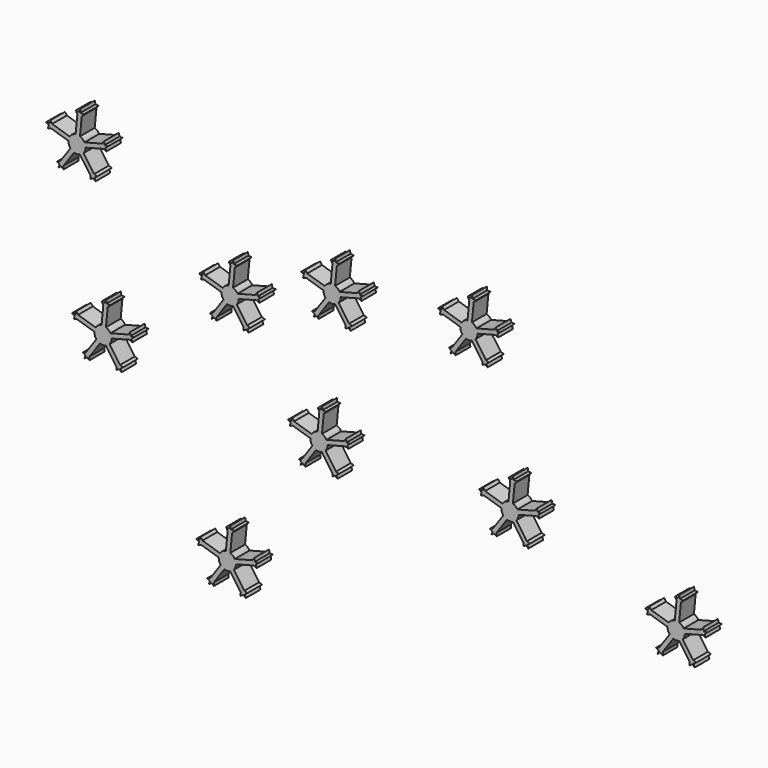
from build123d import *

# Parameters (mm, degrees)
F1_DEPTH = 6.35


# Not quite as in the source:
# - a length typed as a fraction of an inch, garbled in the dataset ("3 / 203.2 mm" for 3/8 in), is restored
# - a feature names something its author has since deleted; it is built from what else it names


with BuildPart() as f1:
    # F0 (on Front) → F1 (new body)
    with BuildSketch(Plane.XZ):
        with BuildLine():
            Line((21.2604275488, -3.1095474934), (20.6556292887, -9.4079404551))
            ThreePointArc((20.6556292887, -9.4079404551), (19.4937557739, -9.8666915905), (18.6236292887, -10.7629519146))
            Line((18.6236292887, -10.7629519146), (12.576675601, -8.900188931))
            Line((12.576675601, -8.900188931), (12.1280131248, -10.3566497037))
            Line((12.1280131248, -10.3566497037), (18.1749668126, -12.2194126873))
            ThreePointArc((18.1749668126, -12.2194126873), (18.3341547138, -13.3009294793), (18.8741556679, -14.2514126873))
            Line((18.8741556679, -14.2514126873), (15.2537081429, -19.4406221217))
            Line((15.2537081429, -19.4406221217), (16.5035738394, -20.3126380279))
            Line((16.5035738394, -20.3126380279), (20.1240213644, -15.1234285936))
            ThreePointArc((20.1240213644, -15.1234285936), (21.1400213644, -15.302786315), (22.1560213644, -15.1234285936))
            Line((22.1560213644, -15.1234285936), (25.7764688895, -20.3126380279))
            Line((25.7764688895, -20.3126380279), (27.026334586, -19.4406221217))
            Line((27.026334586, -19.4406221217), (23.4058870609, -14.2514126873))
            ThreePointArc((23.4058870609, -14.2514126873), (23.9249424171, -13.3597811887), (24.107332834, -12.3443212298))
            Line((24.107332834, -12.3443212298), (30.2273350961, -10.7377387866))
            Line((30.2273350961, -10.7377387866), (29.8403759052, -9.2636836369))
            Line((29.8403759052, -9.2636836369), (23.720373643, -10.87026608))
            ThreePointArc((23.720373643, -10.87026608), (23.0627291406, -10.0753265221), (22.1726513719, -9.5536113146))
            Line((22.1726513719, -9.5536113146), (22.7774496319, -3.2552183529))
            Line((22.7774496319, -3.2552183529), (21.2604275488, -3.1095474934))
        make_face()
        Polygon((12.1280131248, -10.3566497037), (12.576675601, -8.900188931), (11.9083695148, -8.0093797881), (11.5805188378, -9.0736578943), (10.4671907922, -9.0476845099), (11.4021389343, -9.6527018033), (11.0742882573, -10.7169799096), align=None)
        Polygon((20.6949701578, -2.1501670916), (21.2604275488, -3.1095474934), (22.7774496319, -3.2552183529), (23.5151386713, -2.4209715683), (22.4066161069, -2.3145265557), (22.2074849753, -1.2188534252), (21.8034927222, -2.2566121042), align=None)
        Polygon((30.4565886994, -8.3360874916), (29.8403759052, -9.2636836369), (30.2273350961, -10.7377387866), (31.232289885, -11.2175498836), (30.9624783419, -10.1371080538), (31.8394937863, -9.4508160411), (30.7264002425, -9.4165293214), align=None)
        Polygon((28.0786650957, -19.8049719039), (27.026334586, -19.4406221217), (25.7764688895, -20.3126380279), (25.75514866, -21.4260542633), (26.6684530327, -20.7888530485), (27.5300695705, -21.4943792401), (27.165360723, -20.4421731187), align=None)
        Polygon((16.5035738394, -20.3126380279), (15.2537081429, -19.4406221217), (14.2013746901, -19.8049634034), (15.1146790628, -20.4421646183), (14.7499518509, -21.4943643741), (15.6115807023, -20.7888532206), (16.524885075, -21.4260544355), align=None)
    extrude(amount=F1_DEPTH)


with BuildPart() as f1b:
    # F0 (on Front) → F1, piece 2 (new body)
    with BuildSketch(Plane.XZ):
        with BuildLine():
            Line((-25.9454713619, -7.3767473896), (-26.550269622, -13.6751403513))
            ThreePointArc((-26.550269622, -13.6751403513), (-27.7121431369, -14.1338914867), (-28.582269622, -15.0301518109))
            Line((-28.582269622, -15.0301518109), (-34.6292233098, -13.1673888273))
            Line((-34.6292233098, -13.1673888273), (-35.0778857859, -14.6238496))
            Line((-35.0778857859, -14.6238496), (-29.0309320981, -16.4866125836))
            ThreePointArc((-29.0309320981, -16.4866125836), (-28.8717441969, -17.5681293756), (-28.3317432428, -18.5186125836))
            Line((-28.3317432428, -18.5186125836), (-31.9521907679, -23.707822018))
            Line((-31.9521907679, -23.707822018), (-30.7023250714, -24.5798379242))
            Line((-30.7023250714, -24.5798379242), (-27.0818775463, -19.3906284899))
            ThreePointArc((-27.0818775463, -19.3906284899), (-26.0658775463, -19.5699862113), (-25.0498775463, -19.3906284899))
            Line((-25.0498775463, -19.3906284899), (-21.4294300213, -24.5798379242))
            Line((-21.4294300213, -24.5798379242), (-20.1795643248, -23.707822018))
            Line((-20.1795643248, -23.707822018), (-23.8000118498, -18.5186125836))
            ThreePointArc((-23.8000118498, -18.5186125836), (-23.2809564936, -17.6269810849), (-23.0985660768, -16.6115211261))
            Line((-23.0985660768, -16.6115211261), (-16.9785638147, -15.0049386829))
            Line((-16.9785638147, -15.0049386829), (-17.3655230056, -13.5308835331))
            Line((-17.3655230056, -13.5308835331), (-23.4855252677, -15.1374659763))
            ThreePointArc((-23.4855252677, -15.1374659763), (-24.1431697701, -14.3425264184), (-25.0332475389, -13.8208112109))
            Line((-25.0332475389, -13.8208112109), (-24.4284492788, -7.5224182492))
            Line((-24.4284492788, -7.5224182492), (-25.9454713619, -7.3767473896))
        make_face()
        Polygon((-19.1272338151, -24.0721718001), (-20.1795643248, -23.707822018), (-21.4294300213, -24.5798379242), (-21.4507502507, -25.6932541596), (-20.5374458781, -25.0560529447), (-19.6758293402, -25.7615791364), (-20.0405381878, -24.709373015), align=None)
        Polygon((-30.7023250714, -24.5798379242), (-31.9521907679, -23.707822018), (-33.0045242206, -24.0721632997), (-32.0912198479, -24.7093645145), (-32.4559470599, -25.7615642704), (-31.5943182084, -25.0560531169), (-30.6810138358, -25.6932543318), align=None)
        Polygon((-35.0778857859, -14.6238496), (-34.6292233098, -13.1673888273), (-35.2975293959, -12.2765796844), (-35.625380073, -13.3408577906), (-36.7387081186, -13.3148844062), (-35.8037599765, -13.9199016996), (-36.1316106535, -14.9841798058), align=None)
        Polygon((-26.5109287529, -6.4173669878), (-25.9454713619, -7.3767473896), (-24.4284492788, -7.5224182492), (-23.6907602395, -6.6881714645), (-24.7992828039, -6.5817264519), (-24.9984139354, -5.4860533215), (-25.4024061886, -6.5238120004), align=None)
        Polygon((-16.7493102114, -12.6032873879), (-17.3655230056, -13.5308835331), (-16.9785638147, -15.0049386829), (-15.9736090258, -15.4847497799), (-16.2434205689, -14.4043079501), (-15.3664051245, -13.7180159374), (-16.4794986683, -13.6837292177), align=None)
    extrude(amount=F1_DEPTH)


with BuildPart() as f1c:
    # F0 (on Front) → F1, piece 3 (new body)
    with BuildSketch(Plane.XZ):
        with BuildLine():
            Line((-61.1498726017, -19.3782487859), (-61.7546708618, -25.6766417476))
            ThreePointArc((-61.7546708618, -25.6766417476), (-62.9165443766, -26.135392883), (-63.7866708618, -27.0316532072))
            Line((-63.7866708618, -27.0316532072), (-69.8336245495, -25.1688902236))
            Line((-69.8336245495, -25.1688902236), (-70.2822870257, -26.6253509963))
            Line((-70.2822870257, -26.6253509963), (-64.2353333379, -28.4881139799))
            ThreePointArc((-64.2353333379, -28.4881139799), (-64.0761454367, -29.5696307719), (-63.5361444826, -30.5201139799))
            Line((-63.5361444826, -30.5201139799), (-67.1565920076, -35.7093234143))
            Line((-67.1565920076, -35.7093234143), (-65.9067263111, -36.5813393205))
            Line((-65.9067263111, -36.5813393205), (-62.2862787861, -31.3921298862))
            ThreePointArc((-62.2862787861, -31.3921298862), (-61.2702787861, -31.5714876076), (-60.2542787861, -31.3921298862))
            Line((-60.2542787861, -31.3921298862), (-56.633831261, -36.5813393205))
            Line((-56.633831261, -36.5813393205), (-55.3839655645, -35.7093234143))
            Line((-55.3839655645, -35.7093234143), (-59.0044130896, -30.5201139799))
            ThreePointArc((-59.0044130896, -30.5201139799), (-58.4853577334, -29.6284824812), (-58.3029673166, -28.6130225224))
            Line((-58.3029673166, -28.6130225224), (-52.1829650544, -27.0064400792))
            Line((-52.1829650544, -27.0064400792), (-52.5699242453, -25.5323849294))
            Line((-52.5699242453, -25.5323849294), (-58.6899265075, -27.1389673726))
            ThreePointArc((-58.6899265075, -27.1389673726), (-59.3475710099, -26.3440278147), (-60.2376487786, -25.8223126072))
            Line((-60.2376487786, -25.8223126072), (-59.6328505186, -19.5239196455))
            Line((-59.6328505186, -19.5239196455), (-61.1498726017, -19.3782487859))
        make_face()
        Polygon((-51.9537114511, -24.6047887842), (-52.5699242453, -25.5323849294), (-52.1829650544, -27.0064400792), (-51.1780102656, -27.4862511762), (-51.4478218086, -26.4058093464), (-50.5708063642, -25.7195173337), (-51.683899908, -25.685230614), align=None)
        Polygon((-61.7153299927, -18.4188683841), (-61.1498726017, -19.3782487859), (-59.6328505186, -19.5239196455), (-58.8951614792, -18.6896728608), (-60.0036840436, -18.5832278482), (-60.2028151752, -17.4875547178), (-60.6068074283, -18.5253133967), align=None)
        Polygon((-70.2822870257, -26.6253509963), (-69.8336245495, -25.1688902236), (-70.5019306357, -24.2780810807), (-70.8297813127, -25.3423591869), (-71.9431093583, -25.3163858025), (-71.0081612162, -25.9214030959), (-71.3360118933, -26.9856812021), align=None)
        Polygon((-54.3316350549, -36.0736731964), (-55.3839655645, -35.7093234143), (-56.633831261, -36.5813393205), (-56.6551514905, -37.6947555559), (-55.7418471178, -37.057554341), (-54.88023058, -37.7630805327), (-55.2449394275, -36.7108744113), align=None)
        Polygon((-65.9067263111, -36.5813393205), (-67.1565920076, -35.7093234143), (-68.2089254604, -36.073664696), (-67.2956210877, -36.7108659108), (-67.6603482997, -37.7630656667), (-66.7987194482, -37.0575545132), (-65.8854150755, -37.6947557281), align=None)
    extrude(amount=F1_DEPTH)


with BuildPart() as f1d:
    # F0 (on Front) → F1, piece 4 (new body)
    with BuildSketch(Plane.XZ):
        with BuildLine():
            Line((-113.95647353, 9.4253530751), (-114.5612717901, 3.1269601134))
            ThreePointArc((-114.5612717901, 3.1269601134), (-115.723145305, 2.668208978), (-116.5932717901, 1.7719486538))
            Line((-116.5932717901, 1.7719486538), (-122.6402254779, 3.6347116374))
            Line((-122.6402254779, 3.6347116374), (-123.088887954, 2.1782508647))
            Line((-123.088887954, 2.1782508647), (-117.0419342662, 0.3154878811))
            ThreePointArc((-117.0419342662, 0.3154878811), (-116.882746365, -0.7660289109), (-116.3427454109, -1.7165121189))
            Line((-116.3427454109, -1.7165121189), (-119.9631929359, -6.9057215533))
            Line((-119.9631929359, -6.9057215533), (-118.7133272394, -7.7777374595))
            Line((-118.7133272394, -7.7777374595), (-115.0928797144, -2.5885280252))
            ThreePointArc((-115.0928797144, -2.5885280252), (-114.0768797144, -2.7678857466), (-113.0608797144, -2.5885280252))
            Line((-113.0608797144, -2.5885280252), (-109.4404321893, -7.7777374595))
            Line((-109.4404321893, -7.7777374595), (-108.1905664928, -6.9057215533))
            Line((-108.1905664928, -6.9057215533), (-111.8110140179, -1.7165121189))
            ThreePointArc((-111.8110140179, -1.7165121189), (-111.2919586617, -0.8248806202), (-111.1095682449, 0.1905793386))
            Line((-111.1095682449, 0.1905793386), (-104.9895659827, 1.7971617818))
            Line((-104.9895659827, 1.7971617818), (-105.3765251736, 3.2712169316))
            Line((-105.3765251736, 3.2712169316), (-111.4965274358, 1.6646344884))
            ThreePointArc((-111.4965274358, 1.6646344884), (-112.1541719382, 2.4595740463), (-113.044249707, 2.9812892538))
            Line((-113.044249707, 2.9812892538), (-112.4394514469, 9.2796822155))
            Line((-112.4394514469, 9.2796822155), (-113.95647353, 9.4253530751))
        make_face()
        Polygon((-114.521930921, 10.3847334769), (-113.95647353, 9.4253530751), (-112.4394514469, 9.2796822155), (-111.7017624075, 10.1139290002), (-112.8102849719, 10.2203740128), (-113.0094161035, 11.3160471432), (-113.4134083566, 10.2782884643), align=None)
        Polygon((-104.7603123795, 4.1988130768), (-105.3765251736, 3.2712169316), (-104.9895659827, 1.7971617818), (-103.9846111939, 1.3173506848), (-104.254422737, 2.3977925146), (-103.3774072925, 3.0840845273), (-104.4905008364, 3.118371247), align=None)
        Polygon((-123.088887954, 2.1782508647), (-122.6402254779, 3.6347116374), (-123.308531564, 4.5255207803), (-123.636382241, 3.4612426741), (-124.7497102866, 3.4872160585), (-123.8147621445, 2.8821987651), (-124.1426128216, 1.8179206589), align=None)
        Polygon((-118.7133272394, -7.7777374595), (-119.9631929359, -6.9057215533), (-121.0155263887, -7.270062835), (-120.102222016, -7.9072640498), (-120.466949228, -8.9594638057), (-119.6053203765, -8.2539526522), (-118.6920160038, -8.8911538671), align=None)
        Polygon((-107.1382359832, -7.2700713354), (-108.1905664928, -6.9057215533), (-109.4404321893, -7.7777374595), (-109.4617524188, -8.8911536949), (-108.5484480461, -8.25395248), (-107.6868315083, -8.9594786717), (-108.0515403558, -7.9072725503), align=None)
    extrude(amount=F1_DEPTH)


with BuildPart() as f1e:
    # F0 (on Front) → F1, piece 5 (new body)
    with BuildSketch(Plane.XZ):
        with BuildLine():
            Line((-105.0079462535, -45.6497373035), (-105.6127445136, -51.9481302652))
            ThreePointArc((-105.6127445136, -51.9481302652), (-106.7746180284, -52.4068814005), (-107.6447445136, -53.3031417247))
            Line((-107.6447445136, -53.3031417247), (-113.6916982013, -51.4403787411))
            Line((-113.6916982013, -51.4403787411), (-114.1403606775, -52.8968395138))
            Line((-114.1403606775, -52.8968395138), (-108.0934069897, -54.7596024974))
            ThreePointArc((-108.0934069897, -54.7596024974), (-107.9342190885, -55.8411192894), (-107.3942181344, -56.7916024974))
            Line((-107.3942181344, -56.7916024974), (-111.0146656594, -61.9808119318))
            Line((-111.0146656594, -61.9808119318), (-109.7647999629, -62.852827838))
            Line((-109.7647999629, -62.852827838), (-106.1443524379, -57.6636184037))
            ThreePointArc((-106.1443524379, -57.6636184037), (-105.1283524379, -57.8429761251), (-104.1123524379, -57.6636184037))
            Line((-104.1123524379, -57.6636184037), (-100.4919049128, -62.852827838))
            Line((-100.4919049128, -62.852827838), (-99.2420392163, -61.9808119318))
            Line((-99.2420392163, -61.9808119318), (-102.8624867414, -56.7916024974))
            ThreePointArc((-102.8624867414, -56.7916024974), (-102.3434313852, -55.8999709988), (-102.1610409683, -54.8845110399))
            Line((-102.1610409683, -54.8845110399), (-96.0410387062, -53.2779285967))
            Line((-96.0410387062, -53.2779285967), (-96.4279978971, -51.803873447))
            Line((-96.4279978971, -51.803873447), (-102.5480001593, -53.4104558901))
            ThreePointArc((-102.5480001593, -53.4104558901), (-103.2056446617, -52.6155163322), (-104.0957224304, -52.0938011247))
            Line((-104.0957224304, -52.0938011247), (-103.4909241704, -45.795408163))
            Line((-103.4909241704, -45.795408163), (-105.0079462535, -45.6497373035))
        make_face()
        Polygon((-105.5734036445, -44.6903569017), (-105.0079462535, -45.6497373035), (-103.4909241704, -45.795408163), (-102.753235131, -44.9611613784), (-103.8617576954, -44.8547163658), (-104.060888827, -43.7590432353), (-104.4648810801, -44.7968019143), align=None)
        Polygon((-114.1403606775, -52.8968395138), (-113.6916982013, -51.4403787411), (-114.3600042875, -50.5495695982), (-114.6878549645, -51.6138477044), (-115.8011830101, -51.58787432), (-114.866234868, -52.1928916134), (-115.194085545, -53.2571697197), align=None)
        Polygon((-95.8117851029, -50.8762773017), (-96.4279978971, -51.803873447), (-96.0410387062, -53.2779285967), (-95.0360839173, -53.7577396937), (-95.3058954604, -52.6772978639), (-94.428880016, -51.9910058512), (-95.5419735598, -51.9567191315), align=None)
        Polygon((-98.1897087066, -62.345161714), (-99.2420392163, -61.9808119318), (-100.4919049128, -62.852827838), (-100.5132251423, -63.9662440734), (-99.5999207696, -63.3290428586), (-98.7383042318, -64.0345690502), (-99.1030130793, -62.9823629288), align=None)
        Polygon((-109.7647999629, -62.852827838), (-111.0146656594, -61.9808119318), (-112.0669991122, -62.3451532135), (-111.1536947395, -62.9823544284), (-111.5184219514, -64.0345541842), (-110.6567931, -63.3290430307), (-109.7434887273, -63.9662442456), align=None)
    extrude(amount=F1_DEPTH)


with BuildPart() as f1f:
    # F0 (on Front) → F1, piece 6 (new body)
    with BuildSketch(Plane.XZ):
        Polygon((-62.6628538548, -99.3037869547), (-62.0973964638, -100.2631673565), (-60.5803743807, -100.408838216), (-59.8426853414, -99.5745914314), (-60.9512079057, -99.4681464188), (-61.1503390373, -98.3724732883), (-61.5543312905, -99.4102319673), align=None)
        Polygon((-52.9012353133, -105.4897073547), (-53.5174481075, -106.4173035), (-53.1304889165, -107.8913586497), (-52.1255341277, -108.3711697467), (-52.3953456708, -107.2907279169), (-51.5183302264, -106.6044359042), (-52.6314237702, -106.5701491845), align=None)
        Polygon((-55.279158917, -116.9585917669), (-56.3314894267, -116.5942419848), (-57.5813551232, -117.466257891), (-57.6026753526, -118.5796741264), (-56.6893709799, -117.9424729116), (-55.8277544421, -118.6479991032), (-56.1924632897, -117.5957929818), align=None)
        Polygon((-66.8542501732, -117.466257891), (-68.1041158697, -116.5942419848), (-69.1564493225, -116.9585832665), (-68.2431449498, -117.5957844814), (-68.6078721618, -118.6479842372), (-67.7462433103, -117.9424730837), (-66.8329389376, -118.5796742986), align=None)
        with BuildLine():
            Line((-62.0973964638, -100.2631673565), (-62.7021947239, -106.5615603182))
            ThreePointArc((-62.7021947239, -106.5615603182), (-63.8640682388, -107.0203114535), (-64.7341947239, -107.9165717777))
            Line((-64.7341947239, -107.9165717777), (-70.7811484117, -106.0538087941))
            Line((-70.7811484117, -106.0538087941), (-71.2298108878, -107.5102695668))
            Line((-71.2298108878, -107.5102695668), (-65.1828572, -109.3730325504))
            ThreePointArc((-65.1828572, -109.3730325504), (-65.0236692988, -110.4545493424), (-64.4836683447, -111.4050325504))
            Line((-64.4836683447, -111.4050325504), (-68.1041158697, -116.5942419848))
            Line((-68.1041158697, -116.5942419848), (-66.8542501732, -117.466257891))
            Line((-66.8542501732, -117.466257891), (-63.2338026482, -112.2770484567))
            ThreePointArc((-63.2338026482, -112.2770484567), (-62.2178026482, -112.4564061781), (-61.2018026482, -112.2770484567))
            Line((-61.2018026482, -112.2770484567), (-57.5813551232, -117.466257891))
            Line((-57.5813551232, -117.466257891), (-56.3314894267, -116.5942419848))
            Line((-56.3314894267, -116.5942419848), (-59.9519369517, -111.4050325504))
            ThreePointArc((-59.9519369517, -111.4050325504), (-59.4328815955, -110.5134010518), (-59.2504911787, -109.4979410929))
            Line((-59.2504911787, -109.4979410929), (-53.1304889165, -107.8913586497))
            Line((-53.1304889165, -107.8913586497), (-53.5174481075, -106.4173035))
            Line((-53.5174481075, -106.4173035), (-59.6374503696, -108.0238859431))
            ThreePointArc((-59.6374503696, -108.0238859431), (-60.295094872, -107.2289463852), (-61.1851726408, -106.7072311777))
            Line((-61.1851726408, -106.7072311777), (-60.5803743807, -100.408838216))
            Line((-60.5803743807, -100.408838216), (-62.0973964638, -100.2631673565))
        make_face()
        Polygon((-71.2298108878, -107.5102695668), (-70.7811484117, -106.0538087941), (-71.4494544978, -105.1629996512), (-71.7773051749, -106.2272777574), (-72.8906332204, -106.201304373), (-71.9556850783, -106.8063216664), (-72.2835357554, -107.8705997727), align=None)
    extrude(amount=F1_DEPTH)


with BuildPart() as f1g:
    # F0 (on Front) → F1, piece 7 (new body)
    with BuildSketch(Plane.XZ):
        Polygon((-31.0448287009, -52.8231685374), (-30.4793713099, -53.7825489392), (-28.9623492268, -53.9282197987), (-28.2246601875, -53.0939730141), (-29.3331827519, -52.9875280015), (-29.5323138834, -51.891854871), (-29.9363061366, -52.92961355), align=None)
        with BuildLine():
            Line((-30.4793713099, -53.7825489392), (-31.08416957, -60.0809419009))
            ThreePointArc((-31.08416957, -60.0809419009), (-32.2460430849, -60.5396930363), (-33.11616957, -61.4359533604))
            Line((-33.11616957, -61.4359533604), (-39.1631232578, -59.5731903768))
            Line((-39.1631232578, -59.5731903768), (-39.6117857339, -61.0296511496))
            Line((-39.6117857339, -61.0296511496), (-33.5648320461, -62.8924141332))
            ThreePointArc((-33.5648320461, -62.8924141332), (-33.4056441449, -63.9739309251), (-32.8656431908, -64.9244141332))
            Line((-32.8656431908, -64.9244141332), (-36.4860907159, -70.1136235675))
            Line((-36.4860907159, -70.1136235675), (-35.2362250194, -70.9856394738))
            Line((-35.2362250194, -70.9856394738), (-31.6157774943, -65.7964300394))
            ThreePointArc((-31.6157774943, -65.7964300394), (-30.5997774943, -65.9757877608), (-29.5837774943, -65.7964300394))
            Line((-29.5837774943, -65.7964300394), (-25.9633299693, -70.9856394738))
            Line((-25.9633299693, -70.9856394738), (-24.7134642728, -70.1136235675))
            Line((-24.7134642728, -70.1136235675), (-28.3339117978, -64.9244141332))
            ThreePointArc((-28.3339117978, -64.9244141332), (-27.8148564416, -64.0327826345), (-27.6324660248, -63.0173226756))
            Line((-27.6324660248, -63.0173226756), (-21.5124637627, -61.4107402325))
            Line((-21.5124637627, -61.4107402325), (-21.8994229536, -59.9366850827))
            Line((-21.8994229536, -59.9366850827), (-28.0194252157, -61.5432675258))
            ThreePointArc((-28.0194252157, -61.5432675258), (-28.6770697181, -60.748327968), (-29.5671474869, -60.2266127604))
            Line((-29.5671474869, -60.2266127604), (-28.9623492268, -53.9282197987))
            Line((-28.9623492268, -53.9282197987), (-30.4793713099, -53.7825489392))
        make_face()
        Polygon((-21.2832101594, -59.0090889374), (-21.8994229536, -59.9366850827), (-21.5124637627, -61.4107402325), (-20.5075089738, -61.8905513294), (-20.7773205169, -60.8101094996), (-19.9003050725, -60.1238174869), (-21.0133986163, -60.0895307673), align=None)
        Polygon((-23.6611337631, -70.4779733497), (-24.7134642728, -70.1136235675), (-25.9633299693, -70.9856394738), (-25.9846501987, -72.0990557091), (-25.0713458261, -71.4618544943), (-24.2097292882, -72.1673806859), (-24.5744381358, -71.1151745645), align=None)
        Polygon((-35.2362250194, -70.9856394738), (-36.4860907159, -70.1136235675), (-37.5384241686, -70.4779648492), (-36.6251197959, -71.1151660641), (-36.9898470079, -72.1673658199), (-36.1282181564, -71.4618546665), (-35.2149137838, -72.0990558813), align=None)
        Polygon((-39.6117857339, -61.0296511496), (-39.1631232578, -59.5731903768), (-39.8314293439, -58.682381234), (-40.159280021, -59.7466593402), (-41.2726080666, -59.7206859557), (-40.3376599245, -60.3257032492), (-40.6655106015, -61.3899813554), align=None)
    extrude(amount=F1_DEPTH)


with BuildPart() as f1h:
    # F0 (on Front) → F1, piece 8 (new body)
    with BuildSketch(Plane.XZ):
        with BuildLine():
            Line((35.3955293589, -53.5158479562), (34.7907310988, -59.8142409178))
            ThreePointArc((34.7907310988, -59.8142409178), (33.628857584, -60.2729920532), (32.7587310988, -61.1692523774))
            Line((32.7587310988, -61.1692523774), (26.7117774111, -59.3064893938))
            Line((26.7117774111, -59.3064893938), (26.2631149349, -60.7629501665))
            Line((26.2631149349, -60.7629501665), (32.3100686227, -62.6257131501))
            ThreePointArc((32.3100686227, -62.6257131501), (32.4692565239, -63.7072299421), (33.009257478, -64.6577131501))
            Line((33.009257478, -64.6577131501), (29.388809953, -69.8469225845))
            Line((29.388809953, -69.8469225845), (30.6386756495, -70.7189384907))
            Line((30.6386756495, -70.7189384907), (34.2591231745, -65.5297290564))
            ThreePointArc((34.2591231745, -65.5297290564), (35.2751231745, -65.7090867778), (36.2911231745, -65.5297290564))
            Line((36.2911231745, -65.5297290564), (39.9115706996, -70.7189384907))
            Line((39.9115706996, -70.7189384907), (41.1614363961, -69.8469225845))
            Line((41.1614363961, -69.8469225845), (37.540988871, -64.6577131501))
            ThreePointArc((37.540988871, -64.6577131501), (38.0600442272, -63.7660816514), (38.2424346441, -62.7506216926))
            Line((38.2424346441, -62.7506216926), (44.3624369062, -61.1440392494))
            Line((44.3624369062, -61.1440392494), (43.9754777153, -59.6699840997))
            Line((43.9754777153, -59.6699840997), (37.8554754531, -61.2765665428))
            ThreePointArc((37.8554754531, -61.2765665428), (37.1978309507, -60.4816269849), (36.307753182, -59.9599117774))
            Line((36.307753182, -59.9599117774), (36.912551442, -53.6615188157))
            Line((36.912551442, -53.6615188157), (35.3955293589, -53.5158479562))
        make_face()
        Polygon((34.8300719679, -52.5564675543), (35.3955293589, -53.5158479562), (36.912551442, -53.6615188157), (37.6502404814, -52.827272031), (36.541717917, -52.7208270184), (36.3425867854, -51.625153888), (35.9385945323, -52.6629125669), align=None)
        Polygon((44.5916905095, -58.7423879544), (43.9754777153, -59.6699840997), (44.3624369062, -61.1440392494), (45.3673916951, -61.6238503464), (45.097580152, -60.5434085166), (45.9745955964, -59.8571165039), (44.8615020526, -59.8228297842), align=None)
        Polygon((42.2137669058, -70.2112723666), (41.1614363961, -69.8469225845), (39.9115706996, -70.7189384907), (39.8902504701, -71.8323547261), (40.8035548428, -71.1951535112), (41.6651713806, -71.9006797029), (41.3004625331, -70.8484735815), align=None)
        Polygon((30.6386756495, -70.7189384907), (29.388809953, -69.8469225845), (28.3364765002, -70.2112638662), (29.2497808729, -70.848465081), (28.885053661, -71.9006648369), (29.7466825124, -71.1951536834), (30.6599868851, -71.8323548983), align=None)
        Polygon((26.2631149349, -60.7629501665), (26.7117774111, -59.3064893938), (26.0434713249, -58.4156802509), (25.7156206479, -59.4799583571), (24.6022926023, -59.4539849727), (25.5372407444, -60.0590022661), (25.2093900674, -61.1232803723), align=None)
    extrude(amount=F1_DEPTH)


with BuildPart() as f1i:
    # F0 (on Front) → F1, piece 9 (new body)
    with BuildSketch(Plane.XZ):
        with BuildLine():
            Line((92.7706884735, -71.0059741487), (92.1658902134, -77.3043671104))
            ThreePointArc((92.1658902134, -77.3043671104), (91.0040166986, -77.7631182458), (90.1338902134, -78.65937857))
            Line((90.1338902134, -78.65937857), (84.0869365257, -76.7966155863))
            Line((84.0869365257, -76.7966155863), (83.6382740495, -78.2530763591))
            Line((83.6382740495, -78.2530763591), (89.6852277373, -80.1158393427))
            ThreePointArc((89.6852277373, -80.1158393427), (89.8444156385, -81.1973561347), (90.3844165926, -82.1478393427))
            Line((90.3844165926, -82.1478393427), (86.7639690676, -87.3370487771))
            Line((86.7639690676, -87.3370487771), (88.0138347641, -88.2090646833))
            Line((88.0138347641, -88.2090646833), (91.6342822891, -83.0198552489))
            ThreePointArc((91.6342822891, -83.0198552489), (92.6502822891, -83.1992129703), (93.6662822891, -83.0198552489))
            Line((93.6662822891, -83.0198552489), (97.2867298142, -88.2090646833))
            Line((97.2867298142, -88.2090646833), (98.5365955107, -87.3370487771))
            Line((98.5365955107, -87.3370487771), (94.9161479856, -82.1478393427))
            ThreePointArc((94.9161479856, -82.1478393427), (95.4352033418, -81.256207844), (95.6175937587, -80.2407478851))
            Line((95.6175937587, -80.2407478851), (101.7375960208, -78.634165442))
            Line((101.7375960208, -78.634165442), (101.3506368299, -77.1601102922))
            Line((101.3506368299, -77.1601102922), (95.2306345677, -78.7666927354))
            ThreePointArc((95.2306345677, -78.7666927354), (94.5729900653, -77.9717531775), (93.6829122966, -77.4500379699))
            Line((93.6829122966, -77.4500379699), (94.2877105566, -71.1516450082))
            Line((94.2877105566, -71.1516450082), (92.7706884735, -71.0059741487))
        make_face()
        Polygon((92.2052310825, -70.0465937469), (92.7706884735, -71.0059741487), (94.2877105566, -71.1516450082), (95.025399596, -70.3173982236), (93.9168770316, -70.210953211), (93.7177459, -69.1152800805), (93.3137536469, -70.1530387595), align=None)
        Polygon((83.6382740495, -78.2530763591), (84.0869365257, -76.7966155863), (83.4186304395, -75.9058064435), (83.0907797625, -76.9700845497), (81.9774517169, -76.9441111653), (82.912399859, -77.5491284587), (82.584549182, -78.6134065649), align=None)
        Polygon((88.0138347641, -88.2090646833), (86.7639690676, -87.3370487771), (85.7116356148, -87.7013900588), (86.6249399875, -88.3385912736), (86.2602127756, -89.3907910295), (87.121841627, -88.685279876), (88.0351459997, -89.3224810908), align=None)
        Polygon((99.5889260204, -87.7013985592), (98.5365955107, -87.3370487771), (97.2867298142, -88.2090646833), (97.2654095847, -89.3224809187), (98.1787139574, -88.6852797038), (99.0403304952, -89.3908058954), (98.6756216477, -88.3385997741), align=None)
        Polygon((101.9668496241, -76.232514147), (101.3506368299, -77.1601102922), (101.7375960208, -78.634165442), (102.7425508097, -79.1139765389), (102.4727392666, -78.0335347091), (103.349754711, -77.3472426964), (102.2366611672, -77.3129559768), align=None)
    extrude(amount=F1_DEPTH)


solid = Compound([f1.part, f1b.part, f1c.part, f1d.part, f1e.part, f1f.part, f1g.part, f1h.part, f1i.part])
